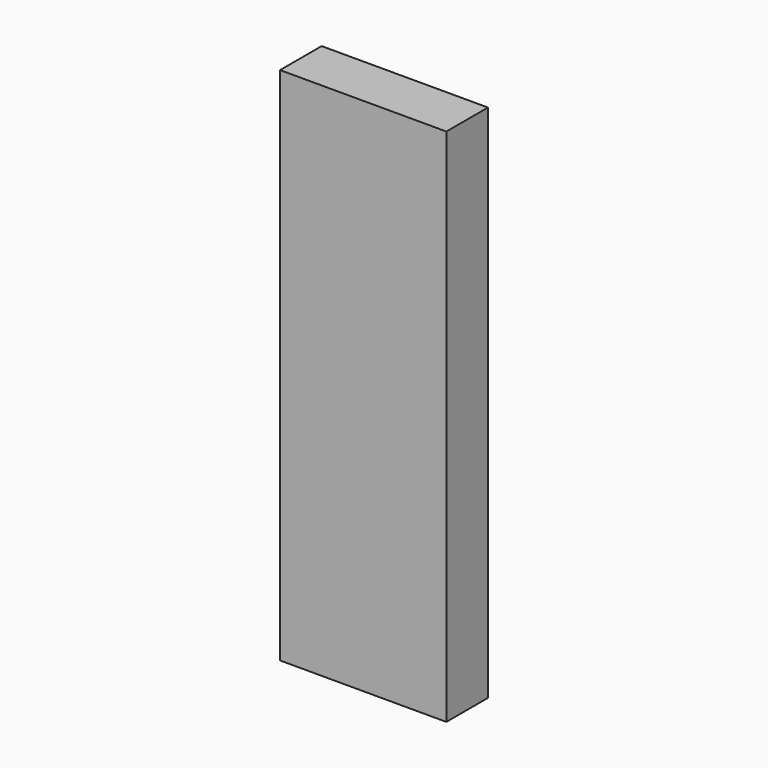
from build123d import *

# Parameters (mm, degrees)
F0_W     = 40.64
F0_H     = 127
F1_DEPTH = 12.7


# Not quite as in the source:
# - a feature names something its author has since deleted; it is built from what else it names


with BuildPart() as f1:
    # F0 (on Front) → F1 (new body)
    with BuildSketch(Plane.XZ):
        Rectangle(F0_W, F0_H)
    extrude(amount=F1_DEPTH)


solid = f1.part
